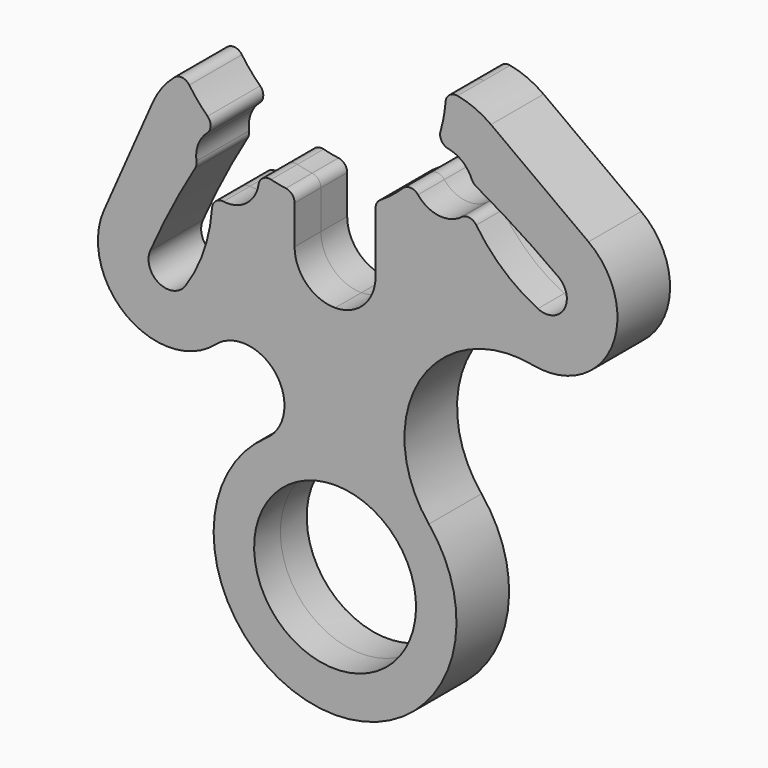
from build123d import *

# Parameters (mm, degrees)
F2_DEPTH = 1.625
F3_R     = 0.5


with BuildPart() as f2:
    # F1 (on Front) → F2 (new body, symmetric)
    with BuildSketch(Plane.XZ):
        with BuildLine():
            Line((-9.013776169, 17.7050338107), (-11.4202907588, 12.2357413908))
            ThreePointArc((-11.4202907588, 12.2357413908), (-10.2877067169, 8.0046358963), (-5.911662711, 8.1923569021))
            ThreePointArc((-5.911662711, 8.1923569021), (-2.9320341736, 7.9056954758), (-3.3935635999, 4.9481032824))
            ThreePointArc((-3.3935635999, 4.9481032824), (-5.7309955372, -1.7764262306), (0, -6))
            ThreePointArc((0, -6), (5.4246164849, -2.5638907917), (4.6360414181, 3.808821336))
            ThreePointArc((4.6360414181, 3.808821336), (4.1819416129, 9.9106242426), (9.7734716353, 12.3951759834))
            ThreePointArc((9.7734716353, 12.3951759834), (13.6570974154, 14.4206268264), (12.5223912203, 18.6511636917))
            Line((12.5223912203, 18.6511636917), (7.703642241, 22.1844525732))
            ThreePointArc((7.703642241, 22.1844525732), (6.6513207463, 22.7390921502), (5.4831457884, 22.9635311317))
            ThreePointArc((5.4831457884, 22.9635311317), (5.3545397461, 21.6786994855), (4.9908089658, 20.4397354858))
            ThreePointArc((4.9908089658, 20.4397354858), (6.1121045533, 20.2513901905), (6.8031849575, 19.3485138867))
            ThreePointArc((6.8031849575, 19.3485138867), (8.9667344033, 18.0591302904), (11.0441073182, 16.6350593529))
            ThreePointArc((11.0441073182, 16.6350593529), (11.3094940429, 15.3128030956), (10.0167213787, 14.9287060214))
            ThreePointArc((10.0167213787, 14.9287060214), (8.0817120955, 16.2654798974), (6.6404774871, 18.1239922393))
            ThreePointArc((6.6404774871, 18.1239922393), (5.1084312653, 17.3870092628), (3.8219991317, 18.4984956094))
            ThreePointArc((3.8219991317, 18.4984956094), (2.9760468043, 17.6620289065), (2, 16.9818491353))
            Line((2, 16.9818491353), (2, 13.7097373258))
            ThreePointArc((2, 13.7097373258), (1.4142135624, 12.2955237634), (0, 11.7097373258))
            ThreePointArc((0, 11.7097373258), (-1.4142135624, 12.2955237634), (-2, 13.7097373258))
            Line((-2, 13.7097373258), (-2, 16.0709631195))
            ThreePointArc((-2, 16.0709631195), (-2.9173667421, 16.2019892223), (-3.809196146, 16.4537229975))
            ThreePointArc((-3.809196146, 16.4537229975), (-3.7756106755, 15.876025127), (-3.9562511801, 15.3262689798))
            ThreePointArc((-3.9562511801, 15.3262689798), (-4.8840043062, 14.5869273446), (-6.0628183167, 14.7201543875))
            ThreePointArc((-6.0628183167, 14.7201543875), (-6.3817079295, 12.3900181819), (-7.3890881873, 10.2648334046))
            ThreePointArc((-7.3890881873, 10.2648334046), (-8.7007106929, 9.9510848963), (-9.1320071762, 11.2288857677))
            ThreePointArc((-9.1320071762, 11.2288857677), (-8.0449849275, 13.5008538339), (-6.8159879432, 15.6992675064))
            ThreePointArc((-6.8159879432, 15.6992675064), (-6.8495734137, 16.2769653768), (-6.6689329091, 16.8267215241))
            ThreePointArc((-6.6689329091, 16.8267215241), (-6.2992442805, 17.2719103955), (-5.7920350927, 17.5504811283))
            ThreePointArc((-5.7920350927, 17.5504811283), (-6.7265171884, 18.4415900362), (-7.4803091112, 19.4899838602))
            ThreePointArc((-7.4803091112, 19.4899838602), (-8.3797588101, 18.7115265217), (-9.013776169, 17.7050338107))
        make_face()
        with BuildLine():
            ThreePointArc((0, -4), (-4, 0), (0, 4))
            ThreePointArc((0, 4), (4, 0), (0, -4))
        make_face(mode=Mode.SUBTRACT)
    extrude(amount=F2_DEPTH, both=True)

    # F3
    f3_edges = [f2.edges().sort_by_distance(p)[0] for p in [
        (-7.480309, 0, 19.489984),
        (-6.815988, -0.8125, 15.699268),
        (-6.815988, 0.8125, 15.699268),
        (-6.062818, -0.8125, 14.720154),
        (-6.062818, 0.8125, 14.720154),
        (2, 0.8125, 16.981849),
        (2, -0.8125, 16.981849),
        (3.821999, -0.8125, 18.498496),
        (3.821999, 0.8125, 18.498496),
        (6.640477, -0.8125, 18.123992),
        (6.640477, 0.8125, 18.123992),
        (4.990809, -0.8125, 20.439735),
        (4.990809, 0.8125, 20.439735),
        (6.803185, -0.8125, 19.348514),
        (6.803185, 0.8125, 19.348514),
        (5.483146, 0.8125, 22.963531),
        (5.483146, -0.8125, 22.963531),
        (-5.792035, 0.8125, 17.550481),
        (-5.792035, -0.8125, 17.550481),
        (-3.809196, 0.8125, 16.453723),
        (-2, 0.8125, 16.070963),
        (-2, -0.8125, 16.070963),
        (-3.809196, -0.8125, 16.453723),
    ]]
    fillet(f3_edges, radius=F3_R)


solid = f2.part
